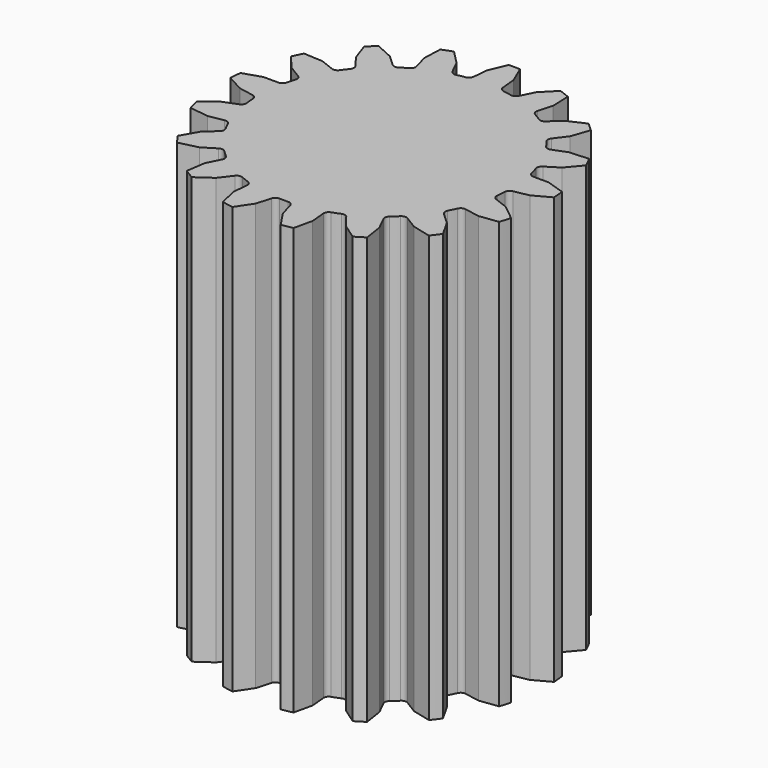
from build123d import *

# Parameters (mm, degrees)
F1_DEPTH = 25
F2_SCALE = 0.6


# Not quite as in the source:
# - ends of sketch curves that miss each other by under 0.0002 mm in the source are joined


with BuildPart() as f1:
    # F0 (on Top) → F1 (new body)
    with BuildSketch(Plane.XY):
        with BuildLine():
            ThreePointArc((7.3874056158, -0.484675036), (7.461653232, -0.3040141279), (7.6313810145, -0.2073520769))
            Line((7.6313810145, -0.2073520769), (8.499995, -0.043795))
            Line((8.499995, -0.043795), (9.484415, 0.490817))
            ThreePointArc((9.484415, 0.490817), (9.45947492, 0.8234317692), (9.4228728682, 1.1549689831))
            Line((9.4228728682, 1.1549689831), (8.356979, 1.499593))
            Line((8.356979, 1.499593), (7.473101, 1.500758))
            ThreePointArc((7.473101, 1.500758), (7.2885019704, 1.5645867929), (7.1823218529, 1.7285289635))
            ThreePointArc((7.1823218529, 1.7285289635), (7.1175094668, 1.9719921552), (7.0444479541, 2.2131049852))
            ThreePointArc((7.0444479541, 2.2131049852), (7.0484187908, 2.4083890769), (7.1717674645, 2.5598368623))
            Line((7.1717674645, 2.5598368623), (7.922642, 3.026128))
            Line((7.922642, 3.026128), (8.647463, 3.880252))
            ThreePointArc((8.647463, 3.880252), (8.5040531833, 4.1813955331), (8.3501576717, 4.4773228219))
            Line((8.3501576717, 4.4773228219), (7.231748, 4.413631))
            Line((7.231748, 4.413631), (6.407136, 4.095424))
            ThreePointArc((6.407136, 4.095424), (6.2119439625, 4.0882570531), (6.0537111889, 4.2027721328))
            ThreePointArc((6.0537111889, 4.2027721328), (5.9053274248, 4.4063813848), (5.750099648, 4.6048195249))
            ThreePointArc((5.750099648, 4.6048195249), (5.6832568969, 4.7883516704), (5.7435669908, 4.9741310069))
            Line((5.7435669908, 4.9741310069), (6.275293, 5.680182))
            Line((6.275293, 5.680182), (6.642623, 6.738465))
            ThreePointArc((6.642623, 6.738465), (6.4001055579, 6.9674725002), (6.1497008123, 7.187822779))
            Line((6.1497008123, 7.187822779), (5.129829, 6.72441))
            Line((5.129829, 6.72441), (4.475851, 6.129807))
            ThreePointArc((4.475851, 6.129807), (4.2964292126, 6.0526130022), (4.1075144193, 6.1022346283))
            ThreePointArc((4.1075144193, 6.1022346283), (3.8955987357, 6.2384913521), (3.6791688772, 6.3674547857))
            ThreePointArc((3.6791688772, 6.3674547857), (3.550540096, 6.5144475711), (3.5396664511, 6.7094678723))
            Line((3.5396664511, 6.7094678723), (3.78043, 7.559923))
            Line((3.78043, 7.559923), (3.74066, 8.679437))
            ThreePointArc((3.74066, 8.679437), (3.4317928439, 8.8053723357), (3.1186980447, 8.9203861287))
            Line((3.1186980447, 8.9203861287), (2.335098, 8.119847))
            Line((2.335098, 8.119847), (1.940078, 7.329152))
            ThreePointArc((1.940078, 7.329152), (1.800657481, 7.1923557065), (1.6065738753, 7.1703824395))
            ThreePointArc((1.6065738753, 7.1703824395), (1.3597445605, 7.2208862875), (1.1113390151, 7.2629580992))
            ThreePointArc((1.1113390151, 7.2629580992), (0.9383027842, 7.3535576382), (0.8577134756, 7.5314809507))
            Line((0.8577134756, 7.5314809507), (0.775, 8.41148))
            Line((0.775, 8.41148), (0.3335, 9.441029))
            ThreePointArc((0.3335, 9.441029), (-1.9988e-06, 9.446885), (-0.3335020113, 9.4410293221))
            Line((-0.3335020113, 9.4410293221), (-0.775, 8.41148))
            Line((-0.775, 8.41148), (-0.857714, 7.531481))
            ThreePointArc((-0.857714, 7.531481), (-0.9383027842, 7.3535576382), (-1.1113430592, 7.2629573897))
            ThreePointArc((-1.1113430592, 7.2629573897), (-1.359747638, 7.2208857122), (-1.606577021, 7.1703820946))
            ThreePointArc((-1.606577021, 7.1703820946), (-1.800657481, 7.1923557065), (-1.9400777424, 7.3291521287))
            Line((-1.9400777424, 7.3291521287), (-2.335099, 8.119847))
            Line((-2.335099, 8.119847), (-3.118701, 8.920385))
            ThreePointArc((-3.118701, 8.920385), (-3.4317963996, 8.8053709582), (-3.7406611723, 8.6794364023))
            Line((-3.7406611723, 8.6794364023), (-3.780431, 7.559923))
            Line((-3.780431, 7.559923), (-3.539666, 6.709468))
            ThreePointArc((-3.539666, 6.709468), (-3.5505402598, 6.5144471694), (-3.6791667182, 6.3674555082))
            ThreePointArc((-3.6791667182, 6.3674555082), (-3.8955977808, 6.2384919434), (-4.1075149705, 6.1022339558))
            ThreePointArc((-4.1075149705, 6.1022339558), (-4.2964292126, 6.0526130022), (-4.4758510731, 6.1298069196))
            Line((-4.4758510731, 6.1298069196), (-5.129829, 6.72441))
            Line((-5.129829, 6.72441), (-6.149704, 7.18782))
            ThreePointArc((-6.149704, 7.18782), (-6.400108148, 6.967470139), (-6.6426230288, 6.7384650295))
            Line((-6.6426230288, 6.7384650295), (-6.275293, 5.680182))
            Line((-6.275293, 5.680182), (-5.743567, 4.974131))
            ThreePointArc((-5.743567, 4.974131), (-5.6832578966, 4.7883516843), (-5.7500984248, 4.6048213441))
            ThreePointArc((-5.7500984248, 4.6048213441), (-5.9053269485, 4.4063820155), (-6.0537118267, 4.2027718781))
            ThreePointArc((-6.0537118267, 4.2027718781), (-6.2119442376, 4.0882569695), (-6.4071360495, 4.0954238717))
            Line((-6.4071360495, 4.0954238717), (-7.231748, 4.413631))
            Line((-7.231748, 4.413631), (-8.350156, 4.477326))
            ThreePointArc((-8.350156, 4.477326), (-8.5040504832, 4.1814009557), (-8.6474626155, 3.8802538251))
            Line((-8.6474626155, 3.8802538251), (-7.922642, 3.026128))
            Line((-7.922642, 3.026128), (-7.171768, 2.559836))
            ThreePointArc((-7.171768, 2.559836), (-7.0484187908, 2.4083890769), (-7.0444474036, 2.2131058081))
            ThreePointArc((-7.0444474036, 2.2131058081), (-7.1175103308, 1.9719891184), (-7.1823216948, 1.7285289243))
            ThreePointArc((-7.1823216948, 1.7285289243), (-7.2885019704, 1.5645867929), (-7.4731020003, 1.50075826))
            Line((-7.4731020003, 1.50075826), (-8.356979, 1.499593))
            Line((-8.356979, 1.499593), (-9.422873, 1.154971))
            ThreePointArc((-9.422873, 1.154971), (-9.4594743605, 0.8234378063), (-9.4844153585, 0.4908200206))
            Line((-9.4844153585, 0.4908200206), (-8.499995, -0.043795))
            Line((-8.499995, -0.043795), (-7.631381, -0.207352))
            ThreePointArc((-7.631381, -0.207352), (-7.461653232, -0.3040141279), (-7.3874056158, -0.484675036))
            ThreePointArc((-7.3874056158, -0.484675036), (-7.3684330117, -0.7358997046), (-7.3409194717, -0.9863359328))
            ThreePointArc((-7.3409194717, -0.9863359328), (-7.3807059844, -1.1775634941), (-7.5297827866, -1.3037675488))
            Line((-7.5297827866, -1.3037675488), (-8.353554, -1.624147))
            Line((-8.353554, -1.624147), (-9.222978, -2.330542))
            ThreePointArc((-9.222978, -2.330542), (-9.1373441946, -2.6529113514), (-9.0404455555, -2.9720778565))
            Line((-9.0404455555, -2.9720778565), (-7.929376, -3.114977))
            Line((-7.929376, -3.114977), (-7.060334, -2.953709))
            ThreePointArc((-7.060334, -2.953709), (-6.8671491722, -2.9825313276), (-6.7326529546, -3.1241709793))
            ThreePointArc((-6.7326529546, -3.1241709793), (-6.6242074857, -3.3515805807), (-6.5080856733, -3.5751628232))
            ThreePointArc((-6.5080856733, -3.5751628232), (-6.4761064028, -3.767850646), (-6.5695260752, -3.9393849177))
            Line((-6.5695260752, -3.9393849177), (-7.221935, -4.53571))
            Line((-7.221935, -4.53571), (-7.77747, -5.508477))
            ThreePointArc((-7.77747, -5.508477), (-7.5811653711, -5.7781417786), (-7.3755138526, -6.0407518803))
            Line((-7.3755138526, -6.0407518803), (-6.287851, -5.772637))
            Line((-6.287851, -5.772637), (-5.53575, -5.308326))
            ThreePointArc((-5.53575, -5.308326), (-5.3451985299, -5.2654149306), (-5.1686181236, -5.3489051266))
            ThreePointArc((-5.1686181236, -5.3489051266), (-4.9853473099, -5.5217814005), (-4.7962997135, -5.6883176634))
            ThreePointArc((-4.7962997135, -5.6883176634), (-4.6968718661, -5.8564426042), (-4.7220182225, -6.0501408896))
            Line((-4.7220182225, -6.0501408896), (-5.114954, -6.841874))
            Line((-5.114954, -6.841874), (-5.28157, -7.949634))
            ThreePointArc((-5.28157, -7.949634), (-5.0011091021, -8.1301755884), (-4.7144791756, -8.3007623071))
            Line((-4.7144791756, -8.3007623071), (-3.797117, -7.657844))
            Line((-3.797117, -7.657844), (-3.263532, -6.953197))
            ThreePointArc((-3.263532, -6.953197), (-3.1013497397, -6.8443476867), (-2.9065329398, -6.858411859))
            ThreePointArc((-2.9065329398, -6.858411859), (-2.6731886588, -6.9534093701), (-2.4367470131, -7.0404080377))
            ThreePointArc((-2.4367470131, -7.0404080377), (-2.28329921, -7.1612630387), (-2.2367755401, -7.3509649507))
            Line((-2.2367755401, -7.3509649507), (-2.31717, -8.231179))
            Line((-2.31717, -8.231179), (-2.072366, -9.324323))
            ThreePointArc((-2.072366, -9.324323), (-1.7456169091, -9.3913601032), (-1.4167189408, -9.4468846077))
            Line((-1.4167189408, -9.4468846077), (-0.793561, -8.515991))
            Line((-0.793561, -8.515991), (-0.550556, -7.666173))
            ThreePointArc((-0.550556, -7.666173), (-0.4386462655, -7.5060887437), (-0.2519050292, -7.4488268576))
            ThreePointArc((-0.2519050292, -7.4488268576), (-1.4991e-06, -7.453115), (0.2519010108, -7.4488263168))
            ThreePointArc((0.2519010108, -7.4488263168), (0.4386457657, -7.50608838), (0.5505559886, -7.6661730033))
            Line((0.5505559886, -7.6661730033), (0.793561, -8.515991))
            Line((0.793561, -8.515991), (1.416723, -9.446884))
            ThreePointArc((1.416723, -9.446884), (1.7456228835, -9.3913589864), (2.0723688731, -9.3243224324))
            Line((2.0723688731, -9.3243224324), (2.317169, -8.231179))
            Line((2.317169, -8.231179), (2.236775, -7.350965))
            ThreePointArc((2.236775, -7.350965), (2.2832994796, -7.1612626201), (2.4367451085, -7.0404093112))
            ThreePointArc((2.4367451085, -7.0404093112), (2.6731892659, -6.953409135), (2.9065358629, -6.8584106789))
            ThreePointArc((2.9065358629, -6.8584106789), (3.1013497397, -6.8443476867), (3.2635328018, -6.9531963929))
            Line((3.2635328018, -6.9531963929), (3.797117, -7.657844))
            Line((3.797117, -7.657844), (4.714475, -8.300765))
            ThreePointArc((4.714475, -8.300765), (5.0011060402, -8.1301774842), (5.281570867, -7.9496338011))
            Line((5.281570867, -7.9496338011), (5.114953, -6.841874))
            Line((5.114953, -6.841874), (4.722018, -6.050141))
            ThreePointArc((4.722018, -6.050141), (4.6968717895, -5.8564429772), (4.7962980952, -5.6883191119))
            ThreePointArc((4.7962980952, -5.6883191119), (4.9853478187, -5.5217809366), (5.1686198468, -5.3489028431))
            ThreePointArc((5.1686198468, -5.3489028431), (5.345198877, -5.2654148922), (5.5357501242, -5.3083257989))
            Line((5.5357501242, -5.3083257989), (6.287851, -5.772637))
            Line((6.287851, -5.772637), (7.375512, -6.040754))
            ThreePointArc((7.375512, -6.040754), (7.5811634373, -5.7781443394), (7.7774690605, -5.5084770424))
            Line((7.7774690605, -5.5084770424), (7.221935, -4.53571))
            Line((7.221935, -4.53571), (6.569526, -3.939385))
            ThreePointArc((6.569526, -3.939385), (6.4761064424, -3.7678508807), (6.508085649, -3.5751633512))
            ThreePointArc((6.508085649, -3.5751633512), (6.6242080803, -3.3515793864), (6.7326532931, -3.1241701337))
            ThreePointArc((6.7326532931, -3.1241701337), (6.8671491722, -2.9825313276), (7.0603338842, -2.9537096242))
            Line((7.0603338842, -2.9537096242), (7.929376, -3.114977))
            Line((7.929376, -3.114977), (9.040445, -2.97208))
            ThreePointArc((9.040445, -2.97208), (9.1373431584, -2.6529149935), (9.2229779242, -2.3305429813))
            Line((9.2229779242, -2.3305429813), (8.353554, -1.624147))
            Line((8.353554, -1.624147), (7.529783, -1.303767))
            ThreePointArc((7.529783, -1.303767), (7.3807060166, -1.1775635483), (7.340919244, -0.986335031))
            ThreePointArc((7.340919244, -0.986335031), (7.3684327304, -0.7359027401), (7.3874056158, -0.484675036))
        make_face()
    extrude(amount=F1_DEPTH)


with BuildPart() as f1_1:
    # F2: moved
    add(f1.part.scale(F2_SCALE))


solid = f1_1.part
